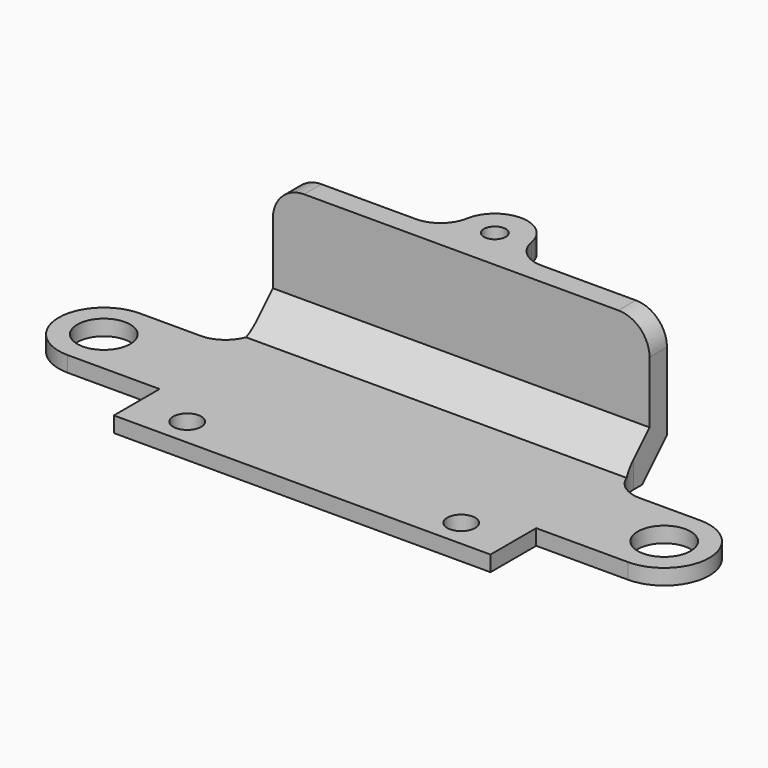
from build123d import *

# Parameters (mm, degrees)
F0_R        = 4.25
F1_DEPTH    = 2.5
F2_W        = 30.2444149011
F2_H        = 3.5
F3_DEPTH    = 19.918
F5_R        = 1.75
F6_DEPTH    = 3
F8_D        = 4.4958
F9_T1_DEPTH = 2.5
F9_T3_DEPTH = 3
F9_T5_DEPTH = 28.5
F10_SIZE    = 5


# Not quite as in the source:
# - a fillet or chamfer that OpenCascade refuses, or shapes differently, is made with other operations: its cross-section is extruded or revolved along the edge and cut away or added


with BuildPart() as f1:
    # F0 (on Top) → F1 (new body)
    with BuildSketch(Plane.XY):
        with BuildLine():
            Line((-30.2444149011, 7.25), (-45, 7.25))
            ThreePointArc((-45, 7.25), (-52.25, 0), (-45, -7.25))
            Line((-45, -7.25), (-30.2444149011, -7.25))
            Line((-30.2444149011, -7.25), (-30.2444149011, -16.4255911708))
            Line((-30.2444149011, -16.4255911708), (0, -16.4255911708))
            Line((0, -16.4255911708), (0, 19))
            Line((0, 19), (-30.2444149011, 19))
            Line((-30.2444149011, 19), (-30.2444149011, 7.25))
        make_face()
        with Locations((-45, 0)):
            Circle(F0_R, mode=Mode.SUBTRACT)
    extrude(amount=F1_DEPTH)

    # F2 (on face) → F3 (join)
    with BuildSketch(Plane.XY.offset(2.5)):
        with Locations((-15.1222074506, 17.25)):
            Rectangle(F2_W, F2_H)
    extrude(amount=F3_DEPTH)

    # F4: F1 across plane


with BuildPart() as f1_1:
    add(f1.part)
    add(f1.part.mirror(Plane.YZ))

    # F5 (on face) → F6 (join)
    with BuildSketch(Plane.XY.offset(22.418)):
        with BuildLine():
            ThreePointArc((4.1231056256, 19), (4.9602824786, 20.5300878706), (5.25, 22.25))
            ThreePointArc((5.25, 22.25), (-1.7199121294, 27.2102824786), (-4.1231056256, 19))
            Line((-4.1231056256, 19), (4.1231056256, 19))
        make_face()
        with Locations((0, 22.25)):
            Circle(F5_R, mode=Mode.SUBTRACT)
    extrude(amount=-F6_DEPTH)

    # F8 (through all)
    with Locations(Plane(origin=(0, 0, 0), x_dir=(1, 0, 0), z_dir=(0, 0, -1))):
        with Locations((-22, 12), (22, 12)):
            Hole(F8_D / 2)

    # F9: fillet of radius 5 on 6 edges, made by hand

    # F9_s2 → F9_t1 (join)
    with BuildSketch(Plane.XY):
        with BuildLine():
            ThreePointArc((30.2444149011, 12.25), (31.7088809952, 8.7144660941), (35.2444149011, 7.25))
            Line((35.2444149011, 7.25), (30.2444149011, 7.25))
            Line((30.2444149011, 7.25), (30.2444149011, 12.25))
        make_face()
        with BuildLine():
            ThreePointArc((-35.2444149011, 7.25), (-31.7088809952, 8.7144660941), (-30.2444149011, 12.25))
            Line((-30.2444149011, 12.25), (-30.2444149011, 7.25))
            Line((-30.2444149011, 7.25), (-35.2444149011, 7.25))
        make_face()
    extrude(amount=F9_T1_DEPTH)

    # F9_s4 → F9_t3 (join)
    with BuildSketch(Plane.XY.offset(19.418)):
        with BuildLine():
            ThreePointArc((10.0995049384, 19), (6.8799003573, 20.1745397216), (5.1729171636, 23.1463414634))
            ThreePointArc((5.1729171636, 23.1463414634), (5.0894053491, 20.9614142663), (4.1231056256, 19))
            Line((4.1231056256, 19), (10.0995049384, 19))
        make_face()
        with BuildLine():
            ThreePointArc((-10.0995049384, 19), (-6.8799003573, 20.1745397216), (-5.1729171636, 23.1463414634))
            ThreePointArc((-5.1729171636, 23.1463414634), (-5.0894053491, 20.9614142663), (-4.1231056256, 19))
            Line((-4.1231056256, 19), (-10.0995049384, 19))
        make_face()
    extrude(amount=F9_T3_DEPTH)

    # F9_s6 → F9_t5 (cut)
    with BuildSketch(Plane.XZ.offset(-31.5)):
        with BuildLine():
            ThreePointArc((-30.2444149011, 17.418), (-28.7799488071, 20.9535339059), (-25.2444149011, 22.418))
            Line((-25.2444149011, 22.418), (-30.2444149011, 22.418))
            Line((-30.2444149011, 22.418), (-30.2444149011, 17.418))
        make_face()
        with BuildLine():
            ThreePointArc((25.2444149011, 22.418), (28.7799488071, 20.9535339059), (30.2444149011, 17.418))
            Line((30.2444149011, 17.418), (30.2444149011, 22.418))
            Line((30.2444149011, 22.418), (25.2444149011, 22.418))
        make_face()
    extrude(amount=F9_T5_DEPTH, mode=Mode.SUBTRACT)

    # F10
    f10_edges = [f1_1.edges().sort_by_distance(p)[0] for p in [
        (0, 19, 0),
        (0, 15.5, 2.5),
    ]]
    chamfer(f10_edges, length=F10_SIZE)


solid = f1_1.part
